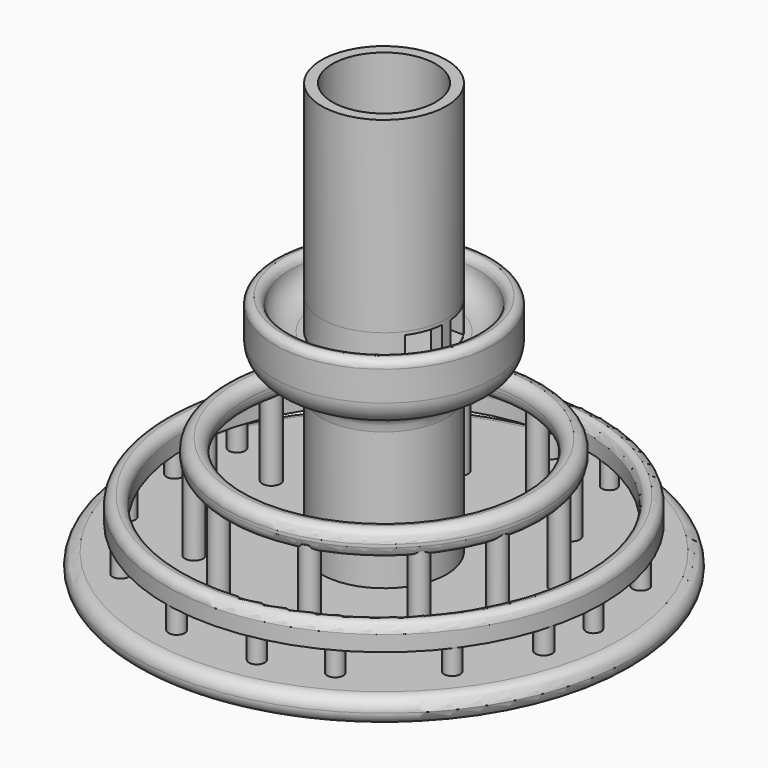
from build123d import *

# Parameters (mm, degrees)
F0_R      = 50.8
F1_DEPTH  = 5.08
F2_R      = 2.53999
F3_R      = 12.7
F4_DEPTH  = 88.9
F6_START  = 38.1
F5_R      = 22.225
F6_DEPTH  = 12.7
F7_R      = 5.08
F8_R      = 19.05
F8_R_2    = 12.7
F9_DEPTH  = 6.35
F10_R     = 5.08
F11_W     = 5.7031868491
F11_H     = 5.6271441281
F11_W_2   = 6.3115260564
F11_H_2   = 5.5511035025
F12_DEPTH = 12.7
F13_W     = 6.40402094
F13_H     = 5.6271441281
F13_W_2   = 5.8219179045
F13_H_2   = 5.6150481105
F14_DEPTH = 12.7
F15_R     = 10.4977096987
F16_DEPTH = 44.45
F17_R     = 1.574799746
F19_START = 20.32
F18_R     = 32.385
F18_R_2   = 27.94
F19_DEPTH = 5.08
F20_R     = 2.22249
F21_R     = 1.8418202524
F22_DEPTH = 21.59
F24_START = 10.16
F23_R     = 44.45
F23_R_2   = 40.64
F24_DEPTH = 5.08
F25_R     = 1.90499
F27_START = 5.08
F26_R     = 1.6477497362
F27_DEPTH = 5.08
F26_R_2   = 1.5192679806
F26_R_3   = 1.6470665841
F26_R_4   = 1.6671776114
F26_R_5   = 1.5508814679
F26_R_6   = 1.7240210591
F26_R_7   = 1.6152426744
F28_R     = 5.08


# Not quite as in the source:
# - a fillet or chamfer is up to 0.001 mm smaller than in the source, because OpenCascade refuses the exact size


with BuildPart() as f1:
    # F0 (on Top) → F1 (new body)
    with BuildSketch(Plane.XY):
        Circle(F0_R)
    extrude(amount=F1_DEPTH)

    # F2 (radius 2.54 in the source; OpenCascade refuses exactly that, so slightly less here)
    f2_edges = [f1.edges().sort_by_distance(p)[0] for p in [
        (50.8, 0, 2.54),
        (-50.8, 0, 0),
        (-50.8, 0, 5.08),
    ]]
    fillet(f2_edges, radius=F2_R)

    # F3 (on Top) → F4 (join)
    with BuildSketch(Plane.XY):
        Circle(F3_R)
    extrude(amount=F4_DEPTH)

    # F5 (on Top) → F6 (join)
    with BuildSketch(Plane.XY.offset(F6_START)):
        Circle(F5_R)
    extrude(amount=F6_DEPTH)

    # F7
    f7_edges = [f1.edges().sort_by_distance(p)[0] for p in [
        (-22.225, 0, 38.1),
    ]]
    fillet(f7_edges, radius=F7_R)

    # F8 (on face) → F9 (cut)
    with BuildSketch(Plane.XY.offset(50.8)):
        Circle(F8_R)
        Circle(F8_R_2, mode=Mode.SUBTRACT)
    extrude(amount=-F9_DEPTH, mode=Mode.SUBTRACT)

    # F10
    f10_edges = [f1.edges().sort_by_distance(p)[0] for p in [
        (-19.05, 0, 44.45),
    ]]
    fillet(f10_edges, radius=F10_R)

    # F11 (on Right) → F12 (cut)
    with BuildSketch(Plane.YZ):
        with Locations((-5.325405742, 47.4032554775)):
            Rectangle(F11_W, F11_H)
        with Locations((5.2445002366, 47.4412757903)):
            Rectangle(F11_W_2, F11_H_2)
    extrude(amount=-F12_DEPTH, mode=Mode.SUBTRACT)

    # F13 (on Right) → F14 (cut)
    with BuildSketch(Plane.YZ):
        with Locations((-4.3034976698, 47.3379362375)):
            Rectangle(F13_W, F13_H)
        with Locations((3.9530118229, 47.3439842463)):
            Rectangle(F13_W_2, F13_H_2)
    extrude(amount=F14_DEPTH, mode=Mode.SUBTRACT)

    # F15 (on face) → F16 (cut)
    with BuildSketch(Plane.XY.offset(88.9)):
        Circle(F15_R)
    extrude(amount=-F16_DEPTH, mode=Mode.SUBTRACT)

    # F17
    f17_edges = [f1.edges().sort_by_distance(p)[0] for p in [
        (-19.05, 0, 50.8),
        (-22.225, 0, 50.8),
    ]]
    fillet(f17_edges, radius=F17_R)

    # F28
    f28_edges = [f1.edges().sort_by_distance(p)[0] for p in [
        (-12.7, 0, 38.1),
    ]]
    fillet(f28_edges, radius=F28_R)


with BuildPart() as f19:
    # F18 (on Top) → F19 (new body)
    with BuildSketch(Plane.XY.offset(F19_START)):
        Circle(F18_R)
        Circle(F18_R_2, mode=Mode.SUBTRACT)
    extrude(amount=F19_DEPTH)

    # F20 (radius 2.2225 in the source; OpenCascade refuses exactly that, so slightly less here)
    f20_edges = [f19.edges().sort_by_distance(p)[0] for p in [
        (-27.94, 0, 25.4),
        (-32.385, 0, 25.4),
        (-27.94, 0, 20.32),
        (-32.385, 0, 20.32),
    ]]
    fillet(f20_edges, radius=F20_R)


with BuildPart() as f22:
    # F21 (on Top) → F22 (new body)
    with BuildSketch(Plane.XY):
        with Locations((-11.4090433344, -27.8096720576)):
            Circle(F21_R)
    extrude(amount=F22_DEPTH)


with BuildPart() as f22b:
    # F21 (on Top) → F22, piece 2 (new body)
    with BuildSketch(Plane.XY):
        with Locations((8.1535298377, -29.0949922055)):
            Circle(F21_R)
    extrude(amount=F22_DEPTH)


with BuildPart() as f22c:
    # F21 (on Top) → F22, piece 3 (new body)
    with BuildSketch(Plane.XY):
        with Locations((22.8778347373, -19.703803584)):
            Circle(F21_R)
    extrude(amount=F22_DEPTH)


with BuildPart() as f22d:
    # F21 (on Top) → F22, piece 4 (new body)
    with BuildSketch(Plane.XY):
        with Locations((-22.6929332038, -19.9089368758)):
            Circle(F21_R)
    extrude(amount=F22_DEPTH)


with BuildPart() as f22e:
    # F21 (on Top) → F22, piece 5 (new body)
    with BuildSketch(Plane.XY):
        with Locations((29.2916446924, -7.8023611568)):
            Circle(F21_R)
    extrude(amount=F22_DEPTH)


with BuildPart() as f22f:
    # F21 (on Top) → F22, piece 6 (new body)
    with BuildSketch(Plane.XY):
        with Locations((29.2916446924, 7.8731411513)):
            Circle(F21_R)
    extrude(amount=F22_DEPTH)


with BuildPart() as f22g:
    # F21 (on Top) → F22, piece 7 (new body)
    with BuildSketch(Plane.XY):
        with Locations((19.9004560709, 22.5974460508)):
            Circle(F21_R)
    extrude(amount=F22_DEPTH)


with BuildPart() as f22h:
    # F21 (on Top) → F22, piece 8 (new body)
    with BuildSketch(Plane.XY):
        with Locations((7.9990136437, 29.011256006)):
            Circle(F21_R)
    extrude(amount=F22_DEPTH)


with BuildPart() as f22i:
    # F21 (on Top) → F22, piece 9 (new body)
    with BuildSketch(Plane.XY):
        with Locations((-8.0465003848, 29.1461069137)):
            Circle(F21_R)
    extrude(amount=F22_DEPTH)


with BuildPart() as f22j:
    # F21 (on Top) → F22, piece 10 (new body)
    with BuildSketch(Plane.XY):
        with Locations((-22.7708052844, 19.7549182922)):
            Circle(F21_R)
    extrude(amount=F22_DEPTH)


with BuildPart() as f22k:
    # F21 (on Top) → F22, piece 11 (new body)
    with BuildSketch(Plane.XY):
        with Locations((-29.1846152395, 7.853475865)):
            Circle(F21_R)
    extrude(amount=F22_DEPTH)


with BuildPart() as f22l:
    # F21 (on Top) → F22, piece 12 (new body)
    with BuildSketch(Plane.XY):
        with Locations((-28.4910995079, -9.9379075691)):
            Circle(F21_R)
    extrude(amount=F22_DEPTH)


with BuildPart() as f24:
    # F23 (on Top) → F24 (new body)
    with BuildSketch(Plane.XY.offset(F24_START)):
        Circle(F23_R)
        Circle(F23_R_2, mode=Mode.SUBTRACT)
    extrude(amount=F24_DEPTH)

    # F25 (radius 1.905 in the source; OpenCascade refuses exactly that, so slightly less here)
    f25_edges = [f24.edges().sort_by_distance(p)[0] for p in [
        (-40.64, 0, 15.24),
        (-44.45, 0, 15.24),
    ]]
    fillet(f25_edges, radius=F25_R)


with BuildPart() as f27:
    # F26 (on Top) → F27 (new body)
    with BuildSketch(Plane.XY.offset(F27_START)):
        with Locations((-18.8590642065, 38.0256585777)):
            Circle(F26_R)
    extrude(amount=F27_DEPTH)


with BuildPart() as f27b:
    # F26 (on Top) → F27, piece 2 (new body)
    with BuildSketch(Plane.XY.offset(F27_START)):
        with Locations((0, 42.6014177501)):
            Circle(F26_R)
    extrude(amount=F27_DEPTH)


with BuildPart() as f27c:
    # F26 (on Top) → F27, piece 3 (new body)
    with BuildSketch(Plane.XY.offset(F27_START)):
        with Locations((-33.3156920969, 26.3522081077)):
            Circle(F26_R)
    extrude(amount=F27_DEPTH)


with BuildPart() as f27d:
    # F26 (on Top) → F27, piece 4 (new body)
    with BuildSketch(Plane.XY.offset(F27_START)):
        with Locations((-40.4543168843, 13.2077103481)):
            Circle(F26_R)
    extrude(amount=F27_DEPTH)


with BuildPart() as f27e:
    # F26 (on Top) → F27, piece 5 (new body)
    with BuildSketch(Plane.XY.offset(F27_START)):
        with Locations((-42.5942614675, 0)):
            Circle(F26_R)
    extrude(amount=F27_DEPTH)


with BuildPart() as f27f:
    # F26 (on Top) → F27, piece 6 (new body)
    with BuildSketch(Plane.XY.offset(F27_START)):
        with Locations((-39.2607972026, -16.1574222147)):
            Circle(F26_R)
    extrude(amount=F27_DEPTH)


with BuildPart() as f27g:
    # F26 (on Top) → F27, piece 7 (new body)
    with BuildSketch(Plane.XY.offset(F27_START)):
        with Locations((-27.8016924858, -32.1618244052)):
            Circle(F26_R)
    extrude(amount=F27_DEPTH)


with BuildPart() as f27h:
    # F26 (on Top) → F27, piece 8 (new body)
    with BuildSketch(Plane.XY.offset(F27_START)):
        with Locations((-8.7942685932, -41.7103096843)):
            Circle(F26_R)
    extrude(amount=F27_DEPTH)


with BuildPart() as f27i:
    # F26 (on Top) → F27, piece 9 (new body)
    with BuildSketch(Plane.XY.offset(F27_START)):
        with Locations((19.987757122, -37.3980102661)):
            Circle(F26_R)
    extrude(amount=F27_DEPTH)


with BuildPart() as f27j:
    # F26 (on Top) → F27, piece 10 (new body)
    with BuildSketch(Plane.XY.offset(F27_START)):
        with Locations((34.2061186544, -25.4354966852)):
            Circle(F26_R)
    extrude(amount=F27_DEPTH)


with BuildPart() as f27k:
    # F26 (on Top) → F27, piece 11 (new body)
    with BuildSketch(Plane.XY.offset(F27_START)):
        with Locations((13.8606047258, 39.9330742657)):
            Circle(F26_R_2)
    extrude(amount=F27_DEPTH)


with BuildPart() as f27l:
    # F26 (on Top) → F27, piece 12 (new body)
    with BuildSketch(Plane.XY.offset(F27_START)):
        with Locations((30.1806572825, 29.9172196537)):
            Circle(F26_R_3)
    extrude(amount=F27_DEPTH)


with BuildPart() as f27m:
    # F26 (on Top) → F27, piece 13 (new body)
    with BuildSketch(Plane.XY.offset(F27_START)):
        with Locations((39.2439626157, 16.1881372333)):
            Circle(F26_R_4)
    extrude(amount=F27_DEPTH)


with BuildPart() as f27n:
    # F26 (on Top) → F27, piece 14 (new body)
    with BuildSketch(Plane.XY.offset(F27_START)):
        with Locations((42.593061924, 0)):
            Circle(F26_R_5)
    extrude(amount=F27_DEPTH)


with BuildPart() as f27o:
    # F26 (on Top) → F27, piece 15 (new body)
    with BuildSketch(Plane.XY.offset(F27_START)):
        with Locations((41.1150082946, -10.7694407925)):
            Circle(F26_R_6)
    extrude(amount=F27_DEPTH)


with BuildPart() as f27p:
    # F26 (on Top) → F27, piece 16 (new body)
    with BuildSketch(Plane.XY.offset(F27_START)):
        with Locations((7.5172022916, -41.6963025928)):
            Circle(F26_R_7)
    extrude(amount=F27_DEPTH)


solid = Compound([f1.part, f19.part, f22.part, f22b.part, f22c.part, f22d.part, f22e.part, f22f.part, f22g.part, f22h.part, f22i.part, f22j.part, f22k.part, f22l.part, f24.part, f27.part, f27b.part, f27c.part, f27d.part, f27e.part, f27f.part, f27g.part, f27h.part, f27i.part, f27j.part, f27k.part, f27l.part, f27m.part, f27n.part, f27o.part, f27p.part])
